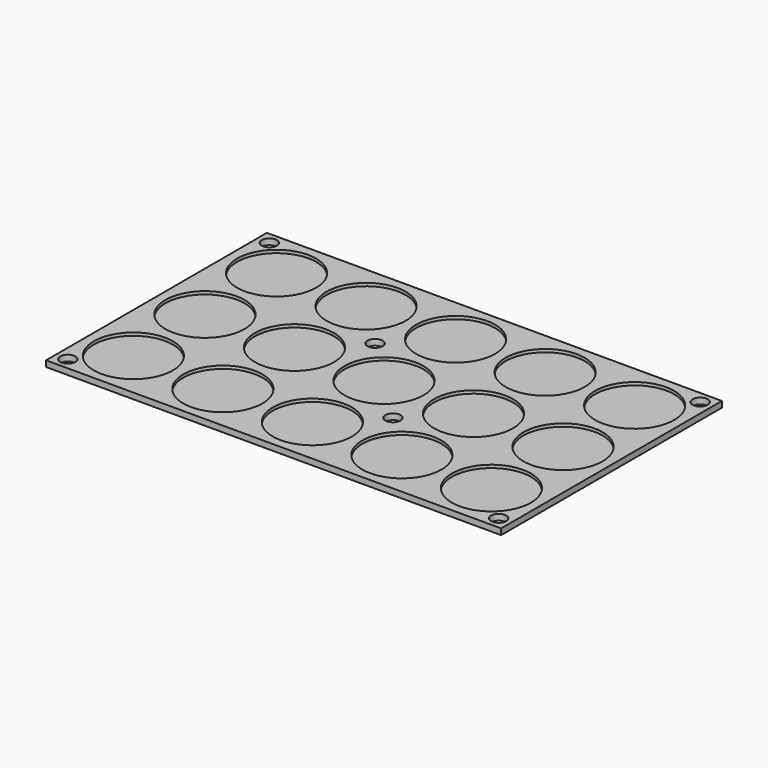
from build123d import *

# Parameters (mm, degrees)
F0_W     = 152.5
F0_H     = 92.5
F0_R     = 13.25
F1_DEPTH = 1
F2_DEPTH = 2
F3_R     = 2.55
F4_DEPTH = 2.001


# Not quite as in the source:
# - a feature names something its author has since deleted; it is built from what else it names


with BuildPart() as f1:
    # F0 (on Top) → F1 (new body)
    with BuildSketch(Plane.XY):
        Rectangle(F0_W, F0_H)
        with Locations((-60, -30)):
            Circle(F0_R, mode=Mode.SUBTRACT)
        with Locations((-30, -30)):
            Circle(F0_R, mode=Mode.SUBTRACT)
        with Locations((0, -30)):
            Circle(F0_R, mode=Mode.SUBTRACT)
        with Locations((30, -30)):
            Circle(F0_R, mode=Mode.SUBTRACT)
        with Locations((60, -30)):
            Circle(F0_R, mode=Mode.SUBTRACT)
        with Locations((-60, 0)):
            Circle(F0_R, mode=Mode.SUBTRACT)
        with Locations((-30, 0)):
            Circle(F0_R, mode=Mode.SUBTRACT)
        with Locations((-60, 30)):
            Circle(F0_R, mode=Mode.SUBTRACT)
        with Locations((-30, 30)):
            Circle(F0_R, mode=Mode.SUBTRACT)
        Circle(F0_R, mode=Mode.SUBTRACT)
        with Locations((30, 0)):
            Circle(F0_R, mode=Mode.SUBTRACT)
        with Locations((60, 0)):
            Circle(F0_R, mode=Mode.SUBTRACT)
        with Locations((0, 30)):
            Circle(F0_R, mode=Mode.SUBTRACT)
        with Locations((30, 30)):
            Circle(F0_R, mode=Mode.SUBTRACT)
        with Locations((60, 30)):
            Circle(F0_R, mode=Mode.SUBTRACT)
        with Locations((-60, 30)):
            Circle(F0_R)
        with Locations((-30, 30)):
            Circle(F0_R)
        with Locations((0, 30)):
            Circle(F0_R)
        with Locations((30, 30)):
            Circle(F0_R)
        with Locations((60, 30)):
            Circle(F0_R)
        with Locations((60, 0)):
            Circle(F0_R)
        with Locations((30, 0)):
            Circle(F0_R)
        with Locations((-30, 0)):
            Circle(F0_R)
        with Locations((-60, 0)):
            Circle(F0_R)
        Circle(F0_R)
        with Locations((0, -30)):
            Circle(F0_R)
        with Locations((-30, -30)):
            Circle(F0_R)
        with Locations((-60, -30)):
            Circle(F0_R)
        with Locations((30, -30)):
            Circle(F0_R)
        with Locations((60, -30)):
            Circle(F0_R)
    extrude(amount=F1_DEPTH)

    # F0 (on Top) → F2 (join)
    with BuildSketch(Plane.XY):
        Rectangle(F0_W, F0_H)
        with Locations((-60, -30)):
            Circle(F0_R, mode=Mode.SUBTRACT)
        with Locations((-30, -30)):
            Circle(F0_R, mode=Mode.SUBTRACT)
        with Locations((0, -30)):
            Circle(F0_R, mode=Mode.SUBTRACT)
        with Locations((30, -30)):
            Circle(F0_R, mode=Mode.SUBTRACT)
        with Locations((60, -30)):
            Circle(F0_R, mode=Mode.SUBTRACT)
        with Locations((-60, 0)):
            Circle(F0_R, mode=Mode.SUBTRACT)
        with Locations((-30, 0)):
            Circle(F0_R, mode=Mode.SUBTRACT)
        with Locations((-60, 30)):
            Circle(F0_R, mode=Mode.SUBTRACT)
        with Locations((-30, 30)):
            Circle(F0_R, mode=Mode.SUBTRACT)
        Circle(F0_R, mode=Mode.SUBTRACT)
        with Locations((30, 0)):
            Circle(F0_R, mode=Mode.SUBTRACT)
        with Locations((60, 0)):
            Circle(F0_R, mode=Mode.SUBTRACT)
        with Locations((0, 30)):
            Circle(F0_R, mode=Mode.SUBTRACT)
        with Locations((30, 30)):
            Circle(F0_R, mode=Mode.SUBTRACT)
        with Locations((60, 30)):
            Circle(F0_R, mode=Mode.SUBTRACT)
    extrude(amount=F2_DEPTH)

    # F3 (on face) → F4 (cut, through all)
    with BuildSketch(Plane.XY.offset(2)):
        with Locations((-72.2, 42.2)):
            Circle(F3_R)
        with Locations((72.2, 42.2)):
            Circle(F3_R)
        with Locations((-72.2, -42.2)):
            Circle(F3_R)
        with Locations((72.2, -42.2)):
            Circle(F3_R)
        with Locations((15, -15)):
            Circle(F3_R)
        with Locations((-15, 15)):
            Circle(F3_R)
    extrude(amount=-F4_DEPTH, mode=Mode.SUBTRACT)


solid = f1.part
